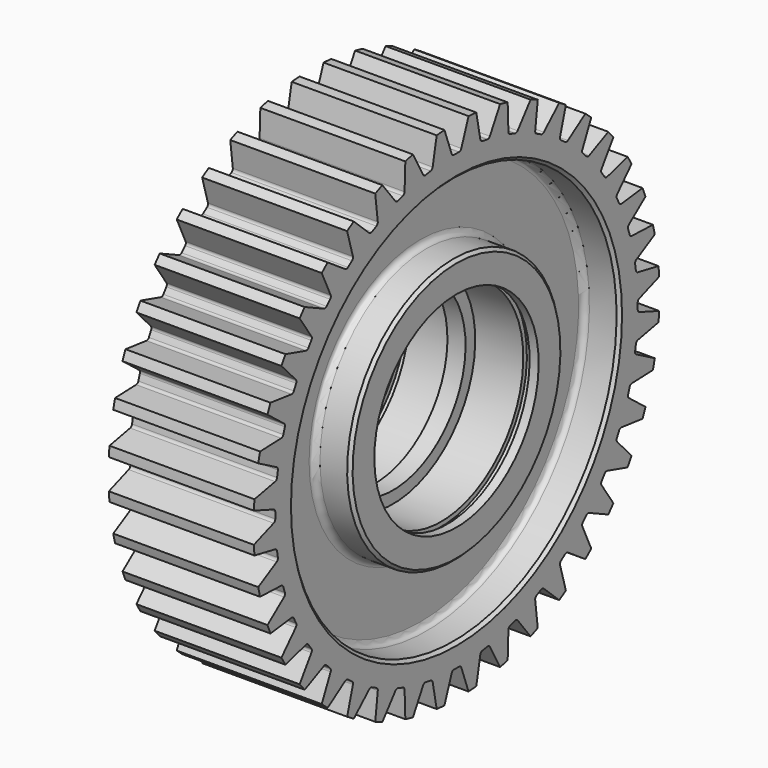
from build123d import *

# Parameters (mm, degrees)
F3_DEPTH = 250
F4_COUNT = 40
F4_ANGLE = 351
F5_SIZE  = 10


with BuildPart() as f1:
    # F0 (on Front) → F1 (revolve)
    with BuildSketch(Plane.XZ):
        with BuildLine():
            Line((240, 840), (0, 840))
            Line((0, 840), (-240, 840))
            Line((-240, 840), (-240, 675))
            Line((-240, 675), (-140, 675))
            ThreePointArc((-140, 675), (-125.8578643763, 669.1421356237), (-120, 655))
            Line((-120, 655), (-120, 460))
            ThreePointArc((-120, 460), (-125.8578643763, 445.8578643763), (-140, 440))
            Line((-140, 440), (-240, 440))
            Line((-240, 440), (-240, 340))
            Line((-240, 340), (-210, 340))
            Line((-210, 340), (-210, 355))
            Line((-210, 355), (-189.0944391489, 355))
            Line((-189.0944391489, 355), (-189.0944391489, 340))
            Line((-189.0944391489, 340), (-30, 340))
            Line((-30, 340), (-30, 300))
            Line((-30, 300), (0, 300))
            Line((0, 300), (30, 300))
            Line((30, 300), (30, 340))
            Line((30, 340), (189.0944391489, 340))
            Line((189.0944391489, 340), (189.0944391489, 355))
            Line((189.0944391489, 355), (210, 355))
            Line((210, 355), (210, 340))
            Line((210, 340), (240, 340))
            Line((240, 340), (240, 440))
            Line((240, 440), (140, 440))
            ThreePointArc((140, 440), (125.8578643763, 445.8578643763), (120, 460))
            Line((120, 460), (120, 655))
            ThreePointArc((120, 655), (125.8578643763, 669.1421356237), (140, 675))
            Line((140, 675), (240, 675))
            Line((240, 675), (240, 840))
        make_face()
    revolve(axis=Axis((-120, 0, 0), (1, 0, 0)))

    # F2 (on Right) → F3 (cut, symmetric)
    with BuildSketch(Plane.YZ):
        with BuildLine():
            ThreePointArc((-10.4128744428, 749.9277112134), (0, 750), (10.4128744428, 749.9277112134))
            ThreePointArc((10.4128744428, 749.9277112134), (16.2304727005, 751.6956061519), (19.9486389765, 756.5065459297))
            Line((19.9486389765, 756.5065459297), (49.8, 838.5224862817))
            ThreePointArc((49.8, 838.5224862817), (0, 840), (-49.8, 838.5224862817))
            Line((-49.8, 838.5224862817), (-19.9486389765, 756.5065459297))
            ThreePointArc((-19.9486389765, 756.5065459297), (-16.2304727005, 751.6956061519), (-10.4128744428, 749.9277112134))
        make_face()
    f3 = extrude(amount=F3_DEPTH, both=True, mode=Mode.SUBTRACT)

    # F4: F3 ×40 about axis
    f4_axis = Axis((240, 0, 0), (-1, 0, 0))
    for i in range(1, F4_COUNT):
        add(f3.rotate(f4_axis, i * F4_ANGLE / (F4_COUNT - 1)), mode=Mode.SUBTRACT)

    # F5
    f5_edges = [f1.edges().sort_by_distance(p)[0] for p in [
        (240, 0, -675),
        (240, 0, -440),
        (-240, 0, -675),
        (-240, 0, -440),
    ]]
    chamfer(f5_edges, length=F5_SIZE)


solid = f1.part
